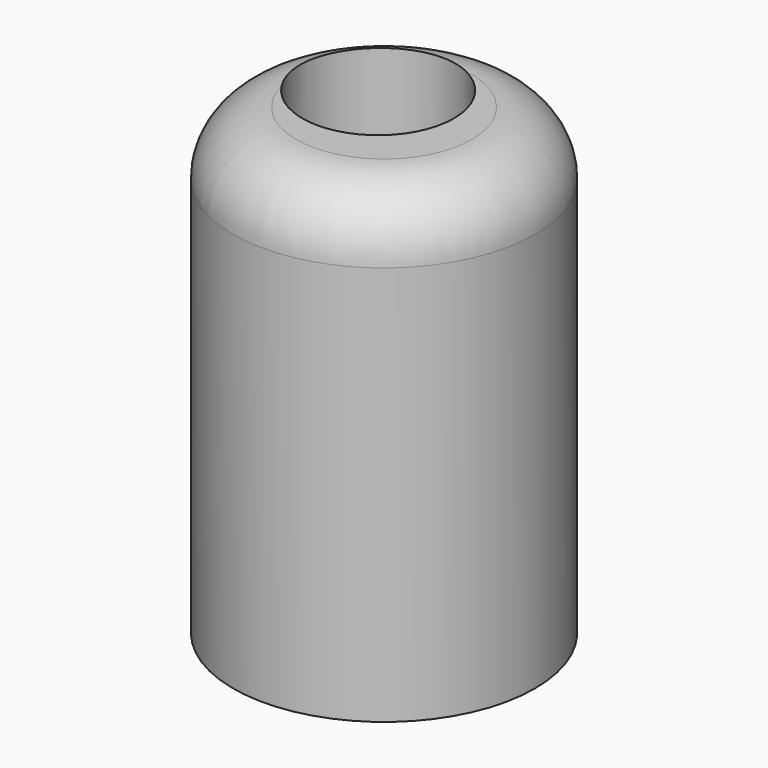
from build123d import *

# Parameters (mm, degrees)
F0_R     = 11.9647327703
F1_DEPTH = 36.7
F2_R     = 6.0094743431
F3_DEPTH = 36.701


# Not quite as in the source:
# - a fillet or chamfer that OpenCascade refuses, or shapes differently, is made with other operations: its cross-section is extruded or revolved along the edge and cut away or added


with BuildPart() as f1:
    # F0 (on Top) → F1 (new body)
    with BuildSketch(Plane.XY):
        Circle(F0_R)
    extrude(amount=F1_DEPTH)

    # F2 (on face) → F3 (cut, through all)
    with BuildSketch(Plane.XY.offset(36.7)):
        with Locations((-1.6841825563, 1.5192364808)):
            Circle(F2_R)
    extrude(amount=-F3_DEPTH, mode=Mode.SUBTRACT)

    # F4: fillet of radius 5 on 1 edges, made by hand

    # F4_s1 → F4_t2 (revolve, cut)
    with BuildSketch(Plane.XZ):
        with BuildLine():
            ThreePointArc((11.9647327703, 31.7), (10.5002666762, 35.2355339059), (6.9647327703, 36.7))
            Line((6.9647327703, 36.7), (11.9647327703, 36.7))
            Line((11.9647327703, 36.7), (11.9647327703, 31.7))
        make_face()
    revolve(axis=Axis((0, 0, 36.7), (0, 0, 1)), mode=Mode.SUBTRACT)


solid = f1.part
